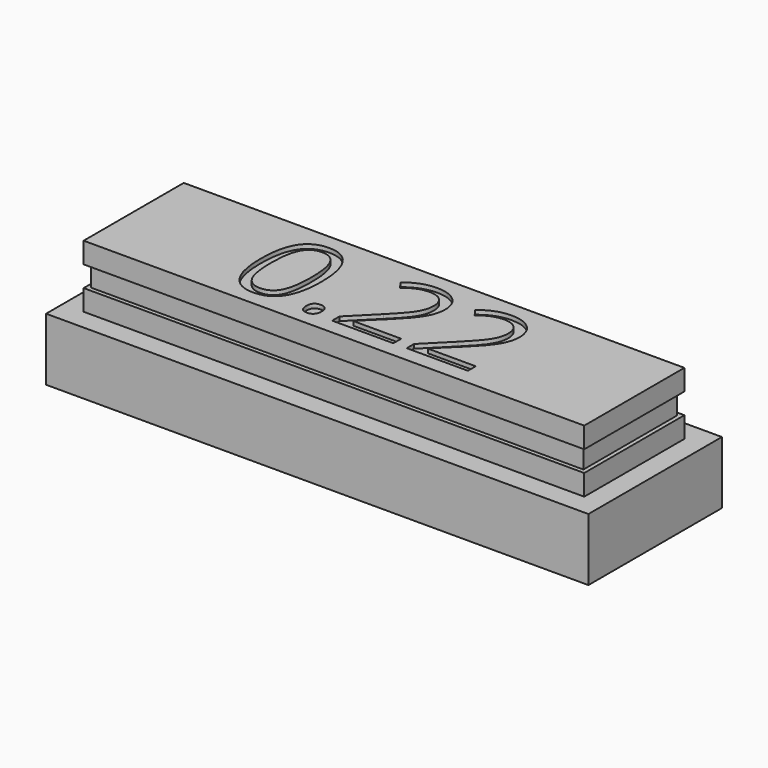
from build123d import *

# Parameters (mm, degrees)
F0_W         = 26
F0_H         = 8
F0_W_2       = 20
F0_H_2       = 2
F1_DEPTH     = 3
F2_W         = 24
F2_H         = 6
F3_DEPTH     = 3
F5_W         = 24
F5_H         = 6
F5_W_2       = 23.6
F5_H_2       = 5.6
F6_DEPTH     = 0.5
F7_W         = 19.56
F7_H         = 1.56
F8_DEPTH     = 3
F9_TEXT_SIZE = 6.25
F10_DEPTH    = 0.2


# Not quite as in the source:
# - Text() gives the source's letters only with a copy of the font that has no kerning and outlines rounded to 1/6400 em; it was checked with that copy


with BuildPart() as f1:
    # F0 (on Top) → F1 (new body)
    with BuildSketch(Plane.XY):
        Rectangle(F0_W, F0_H)
        Rectangle(F0_W_2, F0_H_2, mode=Mode.SUBTRACT)
    extrude(amount=F1_DEPTH)


with BuildPart() as f3:
    # F2 (on face) → F3 (new body)
    with BuildSketch(Plane.XY.offset(3)):
        Rectangle(F2_W, F2_H)
    extrude(amount=F3_DEPTH)

    # F5 (on mid) → F6 (cut, symmetric)
    with BuildSketch(Plane.XY.offset(4.5)):
        Rectangle(F5_W, F5_H)
        Rectangle(F5_W_2, F5_H_2, mode=Mode.SUBTRACT)
    extrude(amount=F6_DEPTH, both=True, mode=Mode.SUBTRACT)

    # F7 (on face) → F8 (join, through all)
    with BuildSketch(Plane(origin=(0, 0, 3), x_dir=(1, 0, 0), z_dir=(0, 0, -1))):
        Rectangle(F7_W, F7_H)
    extrude(amount=F8_DEPTH)

    # F9 (on face) → F10 (cut)
    with BuildSketch(Plane.XY.offset(6)):
        with Locations((-6.2265625, -2.25)):
            Text('0.22', F9_TEXT_SIZE, font='Open Sans', text_align=(TextAlign.LEFT, TextAlign.BOTTOM))
    extrude(amount=-F10_DEPTH, mode=Mode.SUBTRACT)


solid = Compound([f1.part, f3.part])
